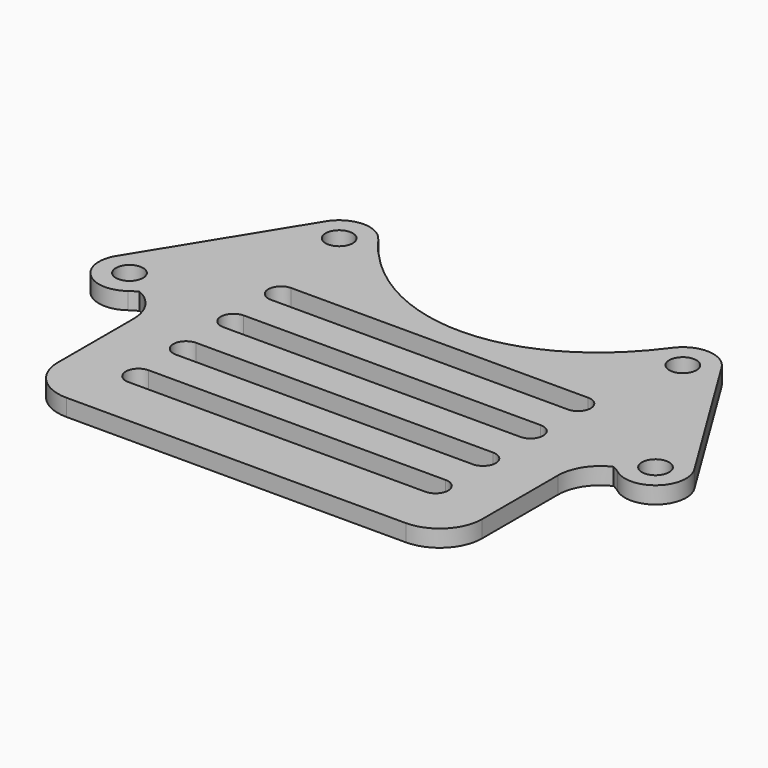
from build123d import *

# Parameters (mm, degrees)
F0_R        = 1.6
F1_DEPTH    = 2
F2_T1_DEPTH = 2
F2_T3_DEPTH = 27
F4_DEPTH    = 25


# Not quite as in the source:
# - a fillet or chamfer that OpenCascade refuses, or shapes differently, is made with other operations: its cross-section is extruded or revolved along the edge and cut away or added


with BuildPart() as f1:
    # F0 (on Top) → F1 (new body)
    with BuildSketch(Plane.XY):
        with BuildLine():
            add(Edge.make_bspline(
                [(-23.1606136078, -2.1185675411), (-22.1073400579, -3.5656171477), (-20.9766129337, -4.8945797394), (-19.7798663886, -6.1017373718)],
                knots=[0, 0, 0, 0, 0.0881031872, 0.0881031872, 0.0881031872, 0.0881031872], degree=3))
            ThreePointArc((-23.1606136078, -2.1185675411), (-23.8473189399, -0.1389116439), (-23.3153209852, 1.887804878))
            Line((-23.3153209852, 1.887804878), (-34.0653209852, -15.5674951767))
            ThreePointArc((-34.0653209852, -15.5674951767), (-32.887804878, -20.5206210399), (-27.9346790148, -19.3431049328))
            Line((-27.9346790148, -19.3431049328), (-19.7798663886, -6.1017373718))
        make_face()
        with Locations((-31, -17.4553000547)):
            Circle(F0_R, mode=Mode.SUBTRACT)
        with BuildLine():
            ThreePointArc((-23.3153209852, 1.887804878), (-23.8473189399, -0.1389116439), (-23.1606136078, -2.1185675411))
            add(Edge.make_bspline(
                [(-23.1606136078, -2.1185675411), (-22.1073400579, -3.5656171477), (-20.9766129337, -4.8945797394), (-19.7798663886, -6.1017373718)],
                knots=[0, 0, 0, 0, 0.0881031872, 0.0881031872, 0.0881031872, 0.0881031872], degree=3))
            Line((-19.7798663886, -6.1017373718), (-17.1846790148, -1.887804878))
            ThreePointArc((-17.1846790148, -1.887804878), (-16.6526810601, 0.1389116439), (-17.3393863922, 2.1185675411))
            ThreePointArc((-17.3393863922, 2.1185675411), (-20.3889116439, 3.5973189399), (-23.3153209852, 1.887804878))
        make_face()
        with Locations((-20.25, 0)):
            Circle(F0_R, mode=Mode.SUBTRACT)
        with BuildLine():
            Line((-17.1846790148, -1.887804878), (-19.7798663886, -6.1017373718))
            add(Edge.make_bspline(
                [(-19.7798663886, -6.1017373718), (-19.2786798287, -6.6072840002), (-17.0287540912, -8.7317983569), (-12.6752714432, -11.7584634521), (-6.4699511651, -14.1622363484), (0, -14.9688818258), (6.4699511651, -14.1622363484), (12.6752714432, -11.7584634521), (17.0287540912, -8.7317983569), (19.2786798287, -6.6072840002), (19.7798663886, -6.1017373718)],
                knots=[0.0881031872, 0.0881031872, 0.0881031872, 0.0881031872, 0.125, 0.25, 0.375, 0.5, 0.625, 0.75, 0.875, 0.9118968128, 0.9118968128, 0.9118968128, 0.9118968128], degree=3))
            Line((19.7798663886, -6.1017373718), (17.1846790148, -1.887804878))
            ThreePointArc((17.1846790148, -1.887804878), (16.6526810601, 0.1389116439), (17.3393863922, 2.1185675411))
            add(Edge.make_bspline(
                [(-17.3393863922, 2.1185675411), (-16.1406178919, 0.4716283513), (-13.5435115335, -2.372660701), (-9.2367539572, -5.3540365479), (-4.6778336966, -7.1127636516), (0, -7.6936181742), (4.6778336966, -7.1127636516), (9.2367539572, -5.3540365479), (13.5435115335, -2.372660701), (16.1406178919, 0.4716283513), (17.3393863922, 2.1185675411)],
                knots=[0, 0, 0, 0, 0.125, 0.25, 0.375, 0.5, 0.625, 0.75, 0.875, 1, 1, 1, 1], degree=3))
            ThreePointArc((-17.3393863922, 2.1185675411), (-16.6526810601, 0.1389116439), (-17.1846790148, -1.887804878))
        make_face()
        with BuildLine():
            add(Edge.make_bspline(
                [(-19.7798663886, -6.1017373718), (-19.2786798287, -6.6072840002), (-17.0287540912, -8.7317983569), (-12.6752714432, -11.7584634521), (-6.4699511651, -14.1622363484), (0, -14.9688818258), (6.4699511651, -14.1622363484), (12.6752714432, -11.7584634521), (17.0287540912, -8.7317983569), (19.2786798287, -6.6072840002), (19.7798663886, -6.1017373718)],
                knots=[0.0881031872, 0.0881031872, 0.0881031872, 0.0881031872, 0.125, 0.25, 0.375, 0.5, 0.625, 0.75, 0.875, 0.9118968128, 0.9118968128, 0.9118968128, 0.9118968128], degree=3))
            Line((-19.7798663886, -6.1017373718), (-27.9346790148, -19.3431049328))
            Line((-27.9346790148, -19.3431049328), (-25, -19.3431049328))
            Line((-25, -19.3431049328), (-25, -40.5))
            Line((-25, -40.5), (0, -40.5))
            Line((0, -40.5), (25, -40.5))
            Line((25, -40.5), (25, -19.3431049328))
            Line((25, -19.3431049328), (27.9346790148, -19.3431049328))
            Line((27.9346790148, -19.3431049328), (19.7798663886, -6.1017373718))
        make_face()
        with BuildLine():
            Line((17.1846790148, -1.887804878), (19.7798663886, -6.1017373718))
            add(Edge.make_bspline(
                [(19.7798663886, -6.1017373718), (20.9766129337, -4.8945797394), (22.1073400579, -3.5656171477), (23.1606136078, -2.1185675411)],
                knots=[0.9118968128, 0.9118968128, 0.9118968128, 0.9118968128, 1, 1, 1, 1], degree=3))
            ThreePointArc((23.1606136078, -2.1185675411), (23.8473189399, -0.1389116439), (23.3153209852, 1.887804878))
            ThreePointArc((23.3153209852, 1.887804878), (20.3889116439, 3.5973189399), (17.3393863922, 2.1185675411))
            ThreePointArc((17.3393863922, 2.1185675411), (16.6526810601, 0.1389116439), (17.1846790148, -1.887804878))
        make_face()
        with Locations((20.25, 0)):
            Circle(F0_R, mode=Mode.SUBTRACT)
        with BuildLine():
            add(Edge.make_bspline(
                [(19.7798663886, -6.1017373718), (20.9766129337, -4.8945797394), (22.1073400579, -3.5656171477), (23.1606136078, -2.1185675411)],
                knots=[0.9118968128, 0.9118968128, 0.9118968128, 0.9118968128, 1, 1, 1, 1], degree=3))
            Line((19.7798663886, -6.1017373718), (27.9346790148, -19.3431049328))
            ThreePointArc((27.9346790148, -19.3431049328), (32.887804878, -20.5206210399), (34.0653209852, -15.5674951767))
            Line((34.0653209852, -15.5674951767), (23.3153209852, 1.887804878))
            ThreePointArc((23.3153209852, 1.887804878), (23.8473189399, -0.1389116439), (23.1606136078, -2.1185675411))
        make_face()
        with Locations((31, -17.4553000547)):
            Circle(F0_R, mode=Mode.SUBTRACT)
    extrude(amount=F1_DEPTH)

    # F2: fillet of radius 5 on 6 edges, made by hand

    # F2_s2 → F2_t1 (join)
    with BuildSketch(Plane.XY):
        with BuildLine():
            ThreePointArc((-25, -24.3431049328), (-26.4644660941, -20.8075710268), (-30, -19.3431049328))
            Line((-30, -19.3431049328), (-25, -19.3431049328))
            Line((-25, -19.3431049328), (-25, -24.3431049328))
        make_face()
        with BuildLine():
            ThreePointArc((-25.8504229337, -19.3431049328), (-27.4279703024, -19.598492799), (-28.8443630885, -20.338567213))
            ThreePointArc((-28.8443630885, -20.338567213), (-28.3424942846, -19.8838105802), (-27.9346790148, -19.3431049328))
            Line((-27.9346790148, -19.3431049328), (-25.8504229337, -19.3431049328))
        make_face()
        with BuildLine():
            ThreePointArc((30, -19.3431049328), (26.4644660941, -20.8075710268), (25, -24.3431049328))
            Line((25, -24.3431049328), (25, -19.3431049328))
            Line((25, -19.3431049328), (30, -19.3431049328))
        make_face()
        with BuildLine():
            ThreePointArc((28.8443630885, -20.338567213), (27.4279703024, -19.598492799), (25.8504229337, -19.3431049328))
            Line((25.8504229337, -19.3431049328), (27.9346790148, -19.3431049328))
            ThreePointArc((27.9346790148, -19.3431049328), (28.3424942846, -19.8838105802), (28.8443630885, -20.338567213))
        make_face()
    extrude(amount=F2_T1_DEPTH)

    # F2_s4 → F2_t3 (cut)
    with BuildSketch(Plane.XY.offset(-12.5)):
        with BuildLine():
            ThreePointArc((-25, -35.5), (-23.5355339059, -39.0355339059), (-20, -40.5))
            Line((-20, -40.5), (-25, -40.5))
            Line((-25, -40.5), (-25, -35.5))
        make_face()
        with BuildLine():
            ThreePointArc((20, -40.5), (23.5355339059, -39.0355339059), (25, -35.5))
            Line((25, -35.5), (25, -40.5))
            Line((25, -40.5), (20, -40.5))
        make_face()
    extrude(amount=F2_T3_DEPTH, mode=Mode.SUBTRACT)

    # F3 (on face) → F4 (cut)
    with BuildSketch(Plane.XY.offset(2)):
        with BuildLine():
            ThreePointArc((-17.5, -10.5), (-19, -12), (-17.5, -13.5))
            Line((-17.5, -13.5), (17.5, -13.5))
            ThreePointArc((17.5, -13.5), (19, -12), (17.5, -10.5))
            Line((17.5, -10.5), (-17.5, -10.5))
        make_face()
        with BuildLine():
            ThreePointArc((-17.5, -17.5), (-19, -19), (-17.5, -20.5))
            Line((-17.5, -20.5), (17.5, -20.5))
            ThreePointArc((17.5, -20.5), (19, -19), (17.5, -17.5))
            Line((17.5, -17.5), (-17.5, -17.5))
        make_face()
        with BuildLine():
            ThreePointArc((-17.5, -24.5), (-19, -26), (-17.5, -27.5))
            Line((-17.5, -27.5), (17.5, -27.5))
            ThreePointArc((17.5, -27.5), (19, -26), (17.5, -24.5))
            Line((17.5, -24.5), (-17.5, -24.5))
        make_face()
        with BuildLine():
            ThreePointArc((-17.5, -31.5), (-19, -33), (-17.5, -34.5))
            Line((-17.5, -34.5), (17.5, -34.5))
            ThreePointArc((17.5, -34.5), (19, -33), (17.5, -31.5))
            Line((17.5, -31.5), (-17.5, -31.5))
        make_face()
    extrude(amount=-F4_DEPTH, mode=Mode.SUBTRACT)


solid = f1.part
